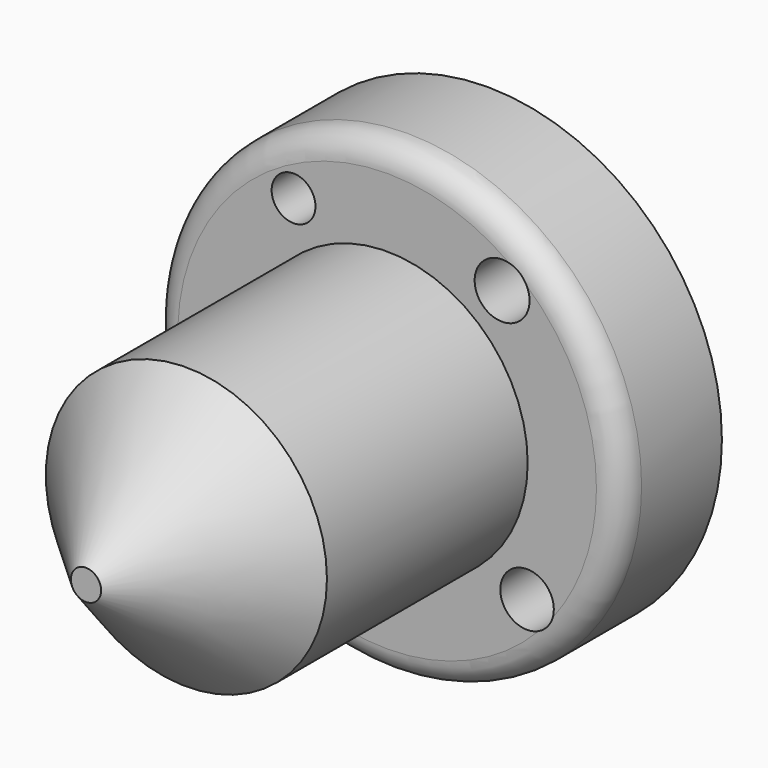
from build123d import *

# Parameters (mm, degrees)
F0_R     = 47.4599930616
F0_R_2   = 5.4133355618
F0_R_3   = 5.4163453987
F0_R_4   = 4.4383518645
F0_R_5   = 28.344153959
F0_R_6   = 5.55874857
F1_DEPTH = 25.4
F2_R     = 28.4576632657
F3_DEPTH = 101.6
F4_SIZE  = 25.4


# Not quite as in the source:
# - a fillet or chamfer that OpenCascade refuses, or shapes differently, is made with other operations: its cross-section is extruded or revolved along the edge and cut away or added


with BuildPart() as f1:
    # F0 (on Front) → F1 (new body)
    with BuildSketch(Plane.XZ):
        Circle(F0_R)
        with Locations((-34.2844575644, -17.503157258)):
            Circle(F0_R_2, mode=Mode.SUBTRACT)
        with Locations((28.3297896385, -24.3600457907)):
            Circle(F0_R_3, mode=Mode.SUBTRACT)
        with Locations((-18.9466699958, 31.7582041025)):
            Circle(F0_R_4, mode=Mode.SUBTRACT)
        Circle(F0_R_5, mode=Mode.SUBTRACT)
        with Locations((23.2773423195, 29.0515273809)):
            Circle(F0_R_6, mode=Mode.SUBTRACT)
    extrude(amount=F1_DEPTH)

    # F2 (on Front) → F3 (join)
    with BuildSketch(Plane.XZ):
        Circle(F2_R)
    extrude(amount=F3_DEPTH)

    # F4
    f4_edges = [f1.edges().sort_by_distance(p)[0] for p in [
        (-28.457663, -101.6, 0),
    ]]
    chamfer(f4_edges, length=F4_SIZE)

    # F5: fillet of radius 5.08 on 1 edges, made by hand

    # F5_s1 → F5_t2 (revolve, cut)
    with BuildSketch(Plane.XY):
        with BuildLine():
            ThreePointArc((42.3799930616, -25.4), (45.9720955101, -23.9121024484), (47.4599930616, -20.32))
            Line((47.4599930616, -20.32), (47.4599930616, -25.4))
            Line((47.4599930616, -25.4), (42.3799930616, -25.4))
        make_face()
    revolve(axis=Axis((0, -25.4, 0), (0, -1, 0)), mode=Mode.SUBTRACT)


solid = f1.part
